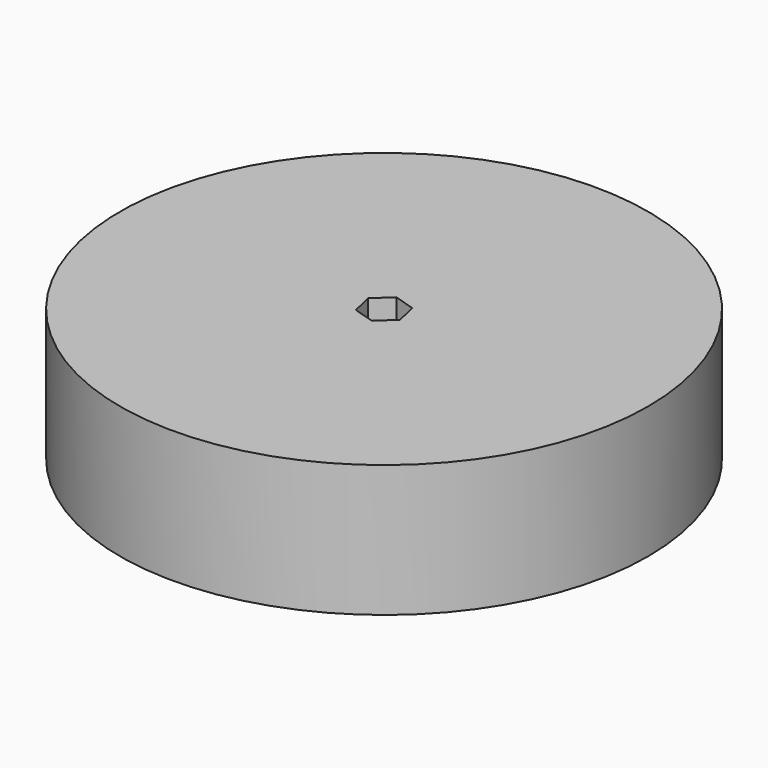
from build123d import *

# Parameters (mm, degrees)
F0_R     = 20
F1_DEPTH = 10
F2_DEPTH = 10


# Not quite as in the source:
# - a feature names something its author has since deleted; it is built from what else it names


with BuildPart() as f1:
    # F0 (on Top) → F1 (new body)
    with BuildSketch(Plane.XY):
        with Locations((31.903732568, 28.4272767603)):
            Circle(F0_R)
        Polygon((33.1302353929, 29.5670241683), (33.5040341896, 27.9349678601), (32.2775313647, 26.7952204522), (30.6772297431, 27.2875293524), (30.3034309464, 28.9195856605), (31.5299337713, 30.0593330685), align=None, mode=Mode.SUBTRACT)
    extrude(amount=F1_DEPTH)

    # F0 (on Top) → F2 (join)
    with BuildSketch(Plane.XY):
        with Locations((31.903732568, 28.4272767603)):
            Circle(F0_R)
        Polygon((33.1302353929, 29.5670241683), (33.5040341896, 27.9349678601), (32.2775313647, 26.7952204522), (30.6772297431, 27.2875293524), (30.3034309464, 28.9195856605), (31.5299337713, 30.0593330685), align=None, mode=Mode.SUBTRACT)
    extrude(amount=F2_DEPTH)


solid = f1.part
